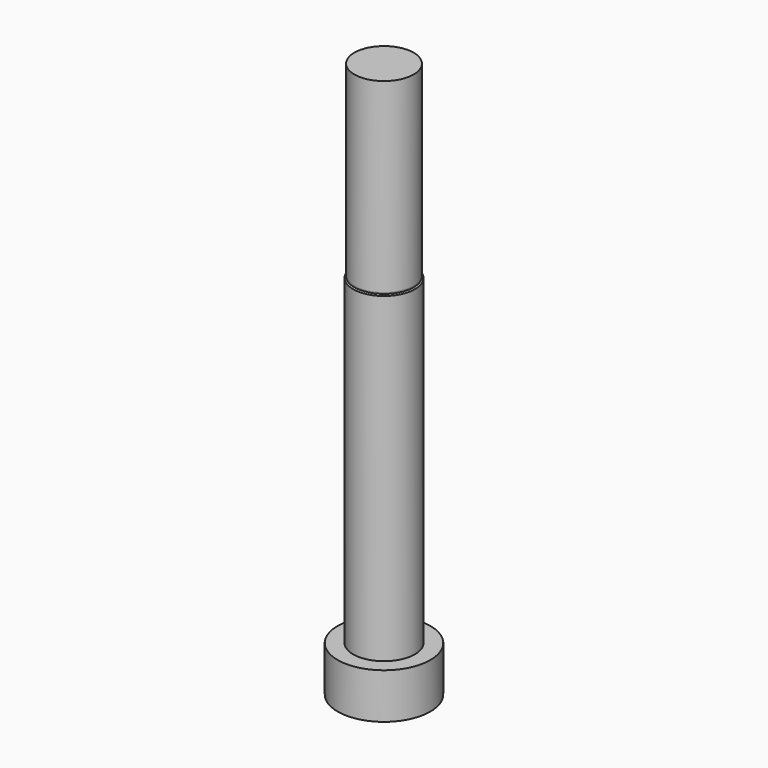
from build123d import *

# Parameters (mm, degrees)
F2_S5_R     = 3.048
F2_T6_DEPTH = 6


# Not quite as in the source:
# - a fillet or chamfer that OpenCascade refuses, or shapes differently, is made with other operations: its cross-section is extruded or revolved along the edge and cut away or added


with BuildPart() as f1:
    # F0 (on Right) → F1 (revolve)
    with BuildSketch(Plane.YZ):
        Polygon((0, 57.15), (0, 0), (4.7625, 0), (4.7625, 4.6736), (3.175, 4.6736), (3.175, 37.9984), (3.048, 37.9984), (3.048, 57.15), align=None)
    revolve(axis=Axis((0, 0, 28.575), (0, 0, -1)))

    # F2: chamfer of 0.254 on 1 edges, made by hand


with BuildPart() as f2_tool2:
    # F2_s3 → F2_t4 (revolve)
    with BuildSketch(Plane.YZ):
        Polygon((3.175, 37.7444), (2.921, 37.9984), (3.175, 37.9984), align=None)
    revolve(axis=Axis((0, 0, 37.9984), (0, 0, -1)))

    # F2_s5 → F2_t6 (cut, symmetric)
    with BuildSketch(Plane.XY.offset(37.9)):
        Circle(F2_S5_R)
    extrude(amount=F2_T6_DEPTH, both=True, mode=Mode.SUBTRACT)


with BuildPart() as f1_1:
    add(f1.part)

    # F2_t1: cut F2_tool2
    add(f2_tool2.part, mode=Mode.SUBTRACT)


solid = f1_1.part
